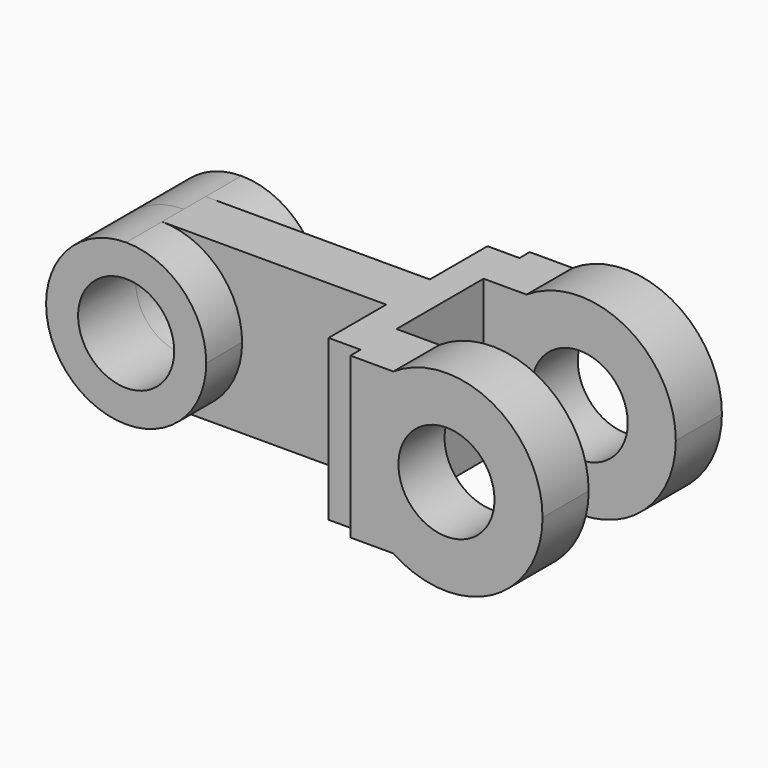
from build123d import *

# Parameters (mm, degrees)
F0_R     = 15
F1_DEPTH = 22.5
F2_DEPTH = 8.5
F3_DEPTH = 31
F5_R     = 15
F6_DEPTH = 18


# Not quite as in the source:
# - a pattern or mirror of a feature is missing from the dataset's text; its kind, count and spacing are read off the source's solid


with BuildPart() as f1:
    # F0 (on Front) → F1 (new body, symmetric)
    with BuildSketch(Plane.XZ):
        with BuildLine():
            ThreePointArc((0, -25), (17.6776695297, -17.6776695297), (25, 0))
            ThreePointArc((25, 0), (17.6776695297, 17.6776695297), (0, 25))
            ThreePointArc((0, 25), (-25, 0), (0, -25))
        make_face()
        Circle(F0_R, mode=Mode.SUBTRACT)
    extrude(amount=F1_DEPTH, both=True)

    # F0 (on Front) → F2 (join, symmetric)
    with BuildSketch(Plane.XZ):
        with BuildLine():
            ThreePointArc((0, 25), (17.6776695297, 17.6776695297), (25, 0))
            ThreePointArc((25, 0), (17.6776695297, -17.6776695297), (0, -25))
            Line((0, -25), (70, -25))
            Line((70, -25), (70, 25))
            Line((70, 25), (0, 25))
        make_face()
    extrude(amount=F2_DEPTH, both=True)

    # F0 (on Front) → F3 (join, symmetric)
    with BuildSketch(Plane.XZ):
        Polygon((80, 25), (70, 25), (70, -25), (80, -25), (80, 0), align=None)
    extrude(amount=F3_DEPTH, both=True)

    # F5 (on offset) → F6 (join)
    with BuildSketch(Plane.XZ.offset(35)):
        with BuildLine():
            ThreePointArc((93.4168760482, -25), (124.1863716546, -26.4338203685), (140, 0))
            ThreePointArc((140, 0), (124.1863716546, 26.4338203685), (93.4168760482, 25))
            ThreePointArc((93.4168760482, 25), (83.5661796315, 14.1863716546), (80, 0))
            ThreePointArc((80, 0), (83.5661796315, -14.1863716546), (93.4168760482, -25))
        make_face()
        with Locations((110, 0)):
            Circle(F5_R, mode=Mode.SUBTRACT)
        with BuildLine():
            ThreePointArc((80, 0), (83.5661796315, 14.1863716546), (93.4168760482, 25))
            Line((93.4168760482, 25), (80, 25))
            Line((80, 25), (80, 0))
        make_face()
        with BuildLine():
            Line((80, -25), (93.4168760482, -25))
            ThreePointArc((93.4168760482, -25), (83.5661796315, -14.1863716546), (80, 0))
            Line((80, 0), (80, -25))
        make_face()
    f6 = extrude(amount=-F6_DEPTH)

    # F6_copies: F6 across plane
    add(f6.mirror(Plane.ZX))


solid = f1.part
